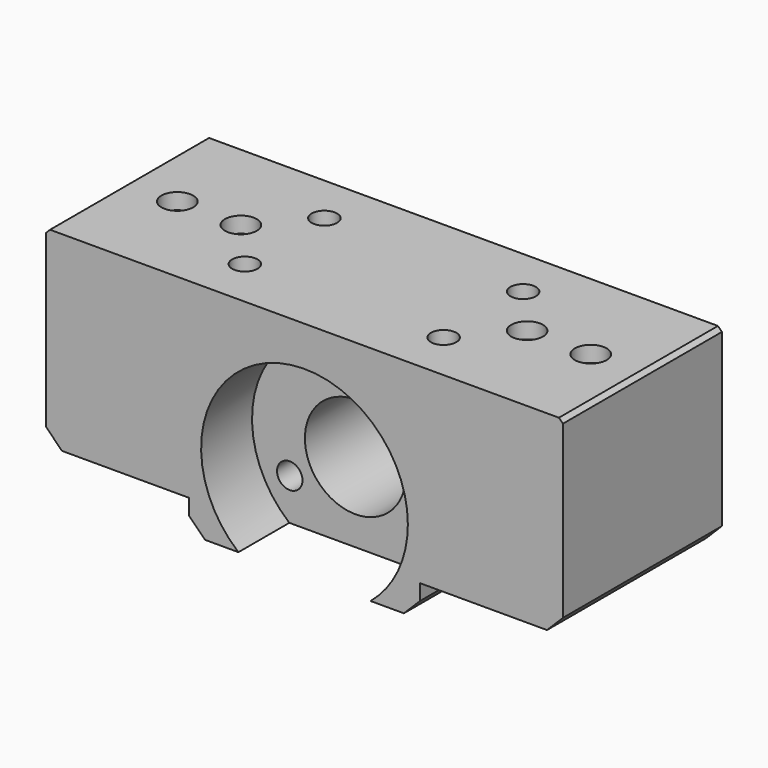
from build123d import *

# Parameters (mm, degrees)
F0_R           = 6.35
F1_DEPTH       = 25
F2_SIZE        = 0.5
F3_R           = 6.35
F4_DEPTH       = 8
F5_SIZE        = 2
F7_D           = 3.2
F7_DEPTH       = 8
F7_TIP         = 0.9613769904
F9_D           = 2.4
F9_CBORE_D     = 4
F9_CBORE_DEPTH = 2
F11_D          = 3.2
F11_DEPTH      = 10
F11_TIP        = 0.9613769904


with BuildPart() as f1:
    # F0 (on Front) → F1 (new body)
    with BuildSketch(Plane.XZ):
        Polygon((-14.5, -10), (14.5, -10), (14.5, -6), (32.5, -6), (32.5, 18), (-32.5, 18), (-32.5, -6), (-14.5, -6), align=None)
        Circle(F0_R, mode=Mode.SUBTRACT)
    extrude(amount=F1_DEPTH)

    # F2
    f2_edges = [f1.edges().sort_by_distance(p)[0] for p in [
        (-32.5, -12.5, 18),
        (32.5, -12.5, 18),
    ]]
    chamfer(f2_edges, length=F2_SIZE)

    # F3 (on face) → F4 (cut)
    with BuildSketch(Plane.XZ.offset(25)):
        with BuildLine():
            ThreePointArc((8.3066238629, -10), (11.7683072321, -5.5233092337), (13, 0))
            ThreePointArc((13, 0), (-5.5233092337, 11.7683072321), (-8.3066238629, -10))
            Line((-8.3066238629, -10), (8.3066238629, -10))
        make_face()
        Circle(F3_R, mode=Mode.SUBTRACT)
    extrude(amount=-F4_DEPTH, mode=Mode.SUBTRACT)

    # F5
    f5_edges = [f1.edges().sort_by_distance(p)[0] for p in [
        (32.5, -12.5, -6),
        (14.5, -12.5, -10),
        (-14.5, -12.5, -10),
        (-32.5, -12.5, -6),
    ]]
    chamfer(f5_edges, length=F5_SIZE)

    # F7
    with Locations(Plane.XY.offset(18)):
        with Locations((12.5, -6.25), (12.5, -18.75), (-12.5, -6.25), (-12.5, -18.75)):
            Hole(F7_D / 2, depth=F7_DEPTH)
            with Locations((0, 0, -(F7_DEPTH + F7_TIP / 2))):  # 118° drill point
                Cone(0, F7_D / 2, F7_TIP, mode=Mode.SUBTRACT)

    # F9 (through all)
    with Locations(Plane.XY.offset(18)):
        with Locations((-26, -12.5), (-18, -12.5), (18, -12.5), (26, -12.5)):
            CounterBoreHole(F9_D / 2, F9_CBORE_D / 2, F9_CBORE_DEPTH)

    # F11
    with Locations(Plane.XZ.offset(17)):
        with Locations((0, 9.53), (8.2532220981, -4.765), (-8.2532220981, -4.765)):
            Hole(F11_D / 2, depth=F11_DEPTH)
            with Locations((0, 0, -(F11_DEPTH + F11_TIP / 2))):  # 118° drill point
                Cone(0, F11_D / 2, F11_TIP, mode=Mode.SUBTRACT)


solid = f1.part
